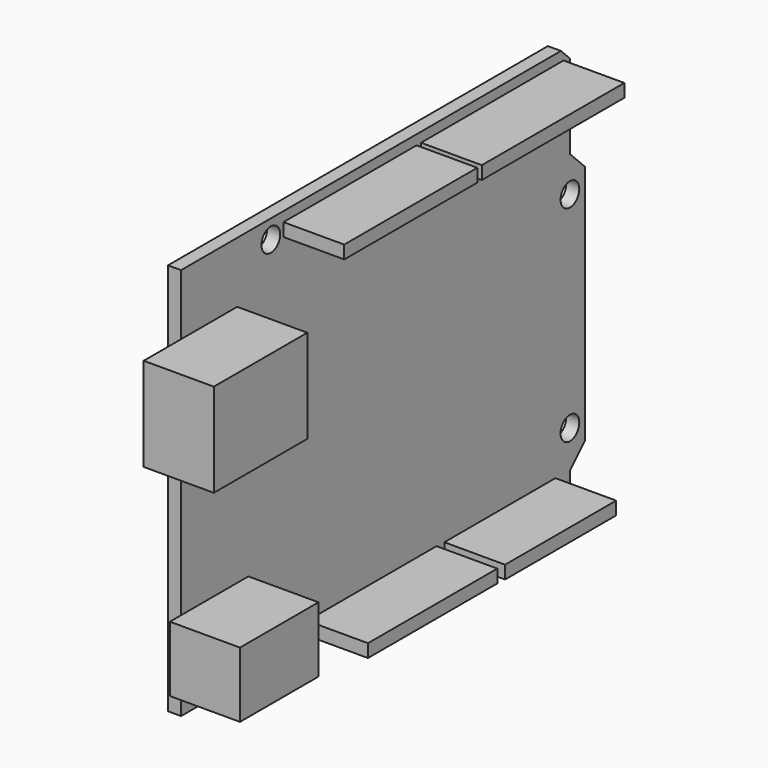
from build123d import *

# Parameters (mm, degrees)
F1_DEPTH = 1.778
F2_R     = 1.5875
F3_DEPTH = 1.778
F4_W     = 13.335
F4_H     = 8.89
F5_DEPTH = 9.525
F4_W_2   = 15.875
F4_H_2   = 12.7
F6_W     = 22.5986149162
F6_H     = 1.778
F7_DEPTH = 8.255
F6_W_2   = 24.2028385401
F6_W_3   = 21.9575874507
F6_W_4   = 18.8628956676


# Not quite as in the source:
# - a feature of the source that left no trace in its solid (it failed there, or was rolled back) is left out


with BuildPart() as f1:
    # F0 (on Right) → F1 (new body)
    with BuildSketch(Plane.YZ):
        Polygon((64.516, 53.34), (0, 53.34), (0, 0), (66.04, 0), (66.04, 2.54), (68.58, 5.08), (68.58, 37.846), (66.04, 40.386), (66.04, 51.816), align=None)
    extrude(amount=F1_DEPTH)

    # F2 (on face) → F3 (cut)
    with BuildSketch(Plane.YZ.offset(1.778)):
        with Locations((13.97, 2.54)):
            Circle(F2_R)
        with Locations((15.24, 50.8)):
            Circle(F2_R)
        with Locations((66.04, 35.56)):
            Circle(F2_R)
        with Locations((66.04, 7.62)):
            Circle(F2_R)
    extrude(amount=-F3_DEPTH, mode=Mode.SUBTRACT)


with BuildPart() as f5:
    # F4 (on face) → F5 (new body)
    with BuildSketch(Plane.YZ.offset(1.778)):
        with Locations((4.7625, 7.62)):
            Rectangle(F4_W, F4_H)
    extrude(amount=F5_DEPTH)


with BuildPart() as f5b:
    # F4 (on face) → F5, piece 2 (new body)
    with BuildSketch(Plane.YZ.offset(1.778)):
        with Locations((1.5875, 38.735)):
            Rectangle(F4_W_2, F4_H_2)
    extrude(amount=F5_DEPTH)


with BuildPart() as f7:
    # F6 (on face) → F7 (new body)
    with BuildSketch(Plane.YZ.offset(1.778)):
        with Locations((28.6866696551, 51.1273522689)):
            Rectangle(F6_W, F6_H)
    extrude(amount=F7_DEPTH)


with BuildPart() as f7b:
    # F6 (on face) → F7, piece 2 (new body)
    with BuildSketch(Plane.YZ.offset(1.778)):
        with Locations((52.8546348214, 51.1273522689)):
            Rectangle(F6_W_2, F6_H)
    extrude(amount=F7_DEPTH)


with BuildPart() as f7c:
    # F6 (on face) → F7, piece 3 (new body)
    with BuildSketch(Plane.YZ.offset(1.778)):
        with Locations((32.4050504714, 1.8045752487)):
            Rectangle(F6_W_3, F6_H)
    extrude(amount=F7_DEPTH)


with BuildPart() as f7d:
    # F6 (on face) → F7, piece 4 (new body)
    with BuildSketch(Plane.YZ.offset(1.778)):
        with Locations((54.1415922344, 1.7308921498)):
            Rectangle(F6_W_4, F6_H)
    extrude(amount=F7_DEPTH)


solid = Compound([f1.part, f5.part, f5b.part, f7.part, f7b.part, f7c.part, f7d.part])
